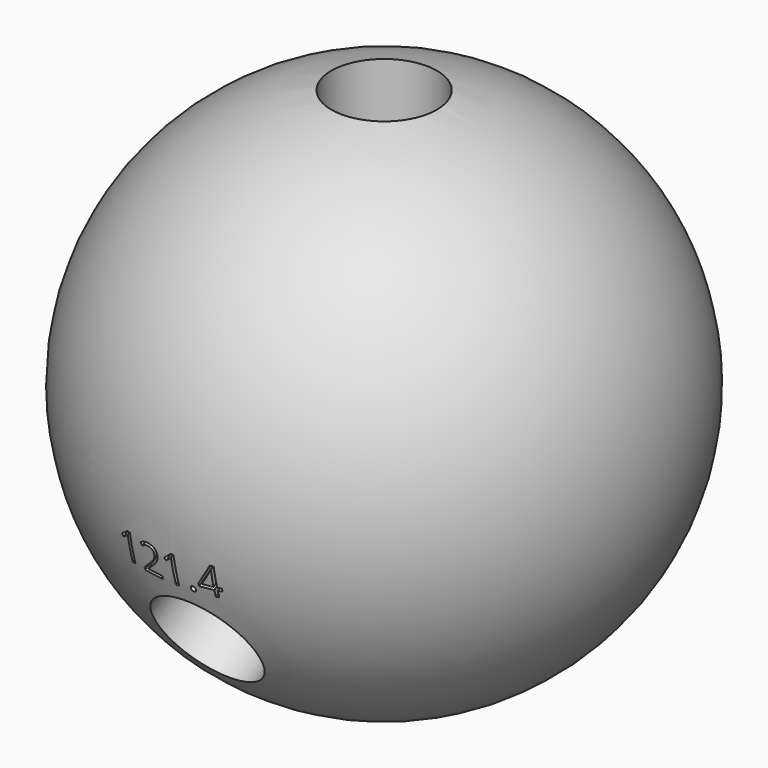
from build123d import *

# Parameters (mm, degrees)
F3_R            = 3.175
F4_DEPTH        = 25.4
F6_ANGLE        = 121.4
F7_ANGLE        = -116.4
F9_TEXT_SIZE    = 3.399471623
F10_DEPTH       = 9.8806
F12_TEXT_SIZE   = 2.4715768329
F12_TEXT_SIZE_2 = 2.0478903833
F13_DEPTH       = 6.6802


# Not quite as in the source:
# - Text() gives the source's letters only with a copy of the font that has no kerning and outlines rounded to 1/6400 em; it was checked with that copy


with BuildPart() as f1:
    # F0 (on Top) → F1 (revolve)
    with BuildSketch(Plane.XY):
        with BuildLine():
            Line((0, -15.875), (0, 15.875))
            ThreePointArc((0, 15.875), (-15.875, 0), (0, -15.875))
        make_face()
    revolve(axis=Axis((0, 0, 0), (0, -1, 0)))

    # F9 (on offset) → F10 (cut)
    with BuildSketch(Plane(origin=(0, 17.0633090326, -8.4703001635), x_dir=(-1, 0, 0), z_dir=(0, 0.8957117602, -0.4446351792))):
        with Locations((-3.8316128775, 7.2181592695)):
            Text('116.4', F9_TEXT_SIZE, font='Open Sans', text_align=(TextAlign.LEFT, TextAlign.BOTTOM))
    extrude(amount=-F10_DEPTH, mode=Mode.SUBTRACT)

    # F12 (on offset) → F13 (cut)
    with BuildSketch(Plane(origin=(0, -16.2601426881, -9.9252334866), x_dir=(1, 0, 0), z_dir=(0, -0.8535507973, -0.5210096318))):
        with Locations((-3.848397173, 4.0336651728)):
            Text('121.4', F12_TEXT_SIZE, font='Open Sans', text_align=(TextAlign.LEFT, TextAlign.BOTTOM))
        with Locations((-3.2727017533, -9.7936345264)):
            Text('122.2', F12_TEXT_SIZE_2, font='Open Sans', text_align=(TextAlign.LEFT, TextAlign.BOTTOM))
    extrude(amount=-F13_DEPTH, mode=Mode.SUBTRACT)


with BuildPart() as f4:
    # F3 (on offset) → F4 (new body)
    with BuildSketch(Plane.XY.offset(6.35)):
        Circle(F3_R)
    extrude(amount=F4_DEPTH)


with BuildPart() as f6_1:
    # F6: copy of F4
    add(f4.part.rotate(Axis((35.7314683497, 0, 0), (1, 0, 0)), F6_ANGLE))


with BuildPart() as f7_1:
    # F7: copy of F4
    add(f4.part.rotate(Axis((35.7314683497, 0, 0), (1, 0, 0)), F7_ANGLE))


with BuildPart() as f1_1:
    add(f1.part)

    # F14: cut F4, F6_1, F7_1
    add(f4.part, mode=Mode.SUBTRACT)
    add(f6_1.part, mode=Mode.SUBTRACT)
    add(f7_1.part, mode=Mode.SUBTRACT)


solid = f1_1.part
